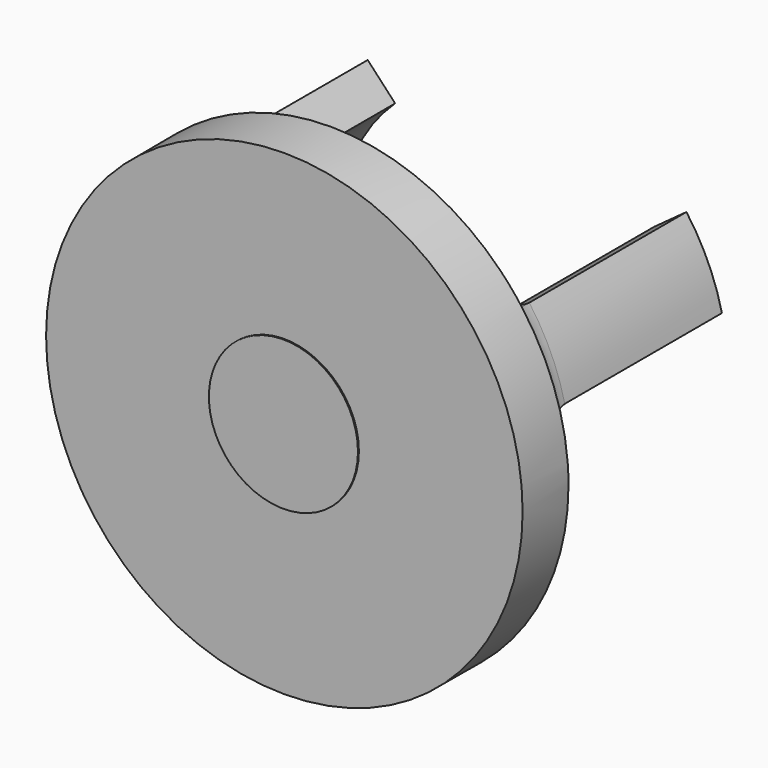
from build123d import *
from build123d import SkipClean  # not in build123d's __all__

# Parameters (mm, degrees)
F0_R          = 6.5
F1_DEPTH      = 0.1
F2_R          = 20.7743809462
F3_DEPTH      = 5
F5_DEPTH      = 25
F6_T4_DEPTH   = 18.5
F6_S5_R       = 18.6353541956
F6_T6_DEPTH   = 12
F6_S7_R       = 15.1353541956
F6_T8_DEPTH   = 12
F6_T10_ANGLE  = 23
F6_T14_DEPTH  = 18.5
F6_S15_R      = 18.6353541956
F6_T16_DEPTH  = 12
F6_S17_R      = 15.1353541956
F6_T18_DEPTH  = 12
F6_T20_ANGLE  = 23
F6_T22_ANGLE  = 23
F6_T26_DEPTH  = 18.5
F6_S27_R      = 18.6353541956
F6_T28_DEPTH  = 12
F6_S29_R      = 15.1353541956
F6_T30_DEPTH  = 12
F6_T32_ANGLE  = 23
F6_T36_DEPTH  = 18.5
F6_S37_R      = 18.6353541956
F6_T38_DEPTH  = 12
F6_S39_R      = 15.1353541956
F6_T40_DEPTH  = 12
F6_T42_ANGLE  = 23
F6_T46_DEPTH  = 18.5
F6_S47_R      = 18.6353541956
F6_T48_DEPTH  = 12
F6_S49_R      = 15.1353541956
F6_T50_DEPTH  = 12
F6_T52_ANGLE  = 23
F6_T56_DEPTH  = 18.5
F6_S57_R      = 18.6353541956
F6_T58_DEPTH  = 11
F6_S59_R      = 15.1353541956
F6_T60_DEPTH  = 11
F6_T65_ANGLE  = 45.0898559736
F6_T69_DEPTH  = 18.5
F6_S70_R      = 20.7743809462
F6_T71_DEPTH  = 12
F6_S72_R      = 18.6353541956
F6_T73_DEPTH  = 12
F6_T79_DEPTH  = 18.5
F6_S80_R      = 15.1353541956
F6_T81_DEPTH  = 12
F6_T84_ANGLE  = 51.3924387562
F6_T91_DEPTH  = 18.5
F6_S92_R      = 15.1353541956
F6_T93_DEPTH  = 12
F6_T96_ANGLE  = 51.3924387562
F6_T103_DEPTH = 18.5
F6_S104_R     = 20.7743809462
F6_T105_DEPTH = 12
F6_S106_R     = 18.6353541956
F6_T107_DEPTH = 12
F6_T110_ANGLE = 45.0898559736
F6_T117_ANGLE = 45.0898559736
F6_T121_DEPTH = 18.5
F6_S122_R     = 20.7743809462
F6_T123_DEPTH = 12
F6_S124_R     = 18.6353541956
F6_T125_DEPTH = 12
F6_T131_ANGLE = 45.0898559736
F6_T135_DEPTH = 18.5
F6_S136_R     = 20.7743809462
F6_T137_DEPTH = 12
F6_S138_R     = 18.6353541956
F6_T139_DEPTH = 12
F6_T145_DEPTH = 18.5
F6_S146_R     = 15.1353541956
F6_T147_DEPTH = 12
F6_T150_ANGLE = 51.3924387562
F6_T157_ANGLE = 51.3924387562
F6_T161_DEPTH = 18.5
F6_S162_R     = 15.1353541956
F6_T163_DEPTH = 12
F6_T169_DEPTH = 18.5
F6_S170_R     = 20.7743809462
F6_T171_DEPTH = 12
F6_S172_R     = 18.6353541956
F6_T173_DEPTH = 12
F6_T176_ANGLE = 45.0898559736
F6_T183_ANGLE = 45.0898559736
F6_T187_DEPTH = 18.5
F6_S188_R     = 20.7743809462
F6_T189_DEPTH = 11
F6_S190_R     = 18.6353541956
F6_T191_DEPTH = 11
F6_T197_DEPTH = 18.5
F6_S198_R     = 15.1353541956
F6_T199_DEPTH = 12
F6_T202_ANGLE = 51.3924387562
F6_T209_DEPTH = 18.5
F6_S210_R     = 15.1353541956
F6_T211_DEPTH = 11
F6_T214_ANGLE = 51.3924387562


# Not quite as in the source:
# - a fillet or chamfer that OpenCascade refuses, or shapes differently, is made with other operations: its cross-section is extruded or revolved along the edge and cut away or added


with BuildPart() as f1:
    # F0 (on Front) → F1 (new body)
    with BuildSketch(Plane.XZ):
        Circle(F0_R)
    extrude(amount=F1_DEPTH)

    # F2 (on Front) → F3 (join)
    with BuildSketch(Plane.XZ):
        Circle(F2_R)
    extrude(amount=-F3_DEPTH)

    # F4 (on face) → F5 (join)
    with BuildSketch(Plane.XZ):
        with BuildLine():
            Line((-10.3406240467, 11.052169061), (-12.7318587476, 13.6079461649))
            ThreePointArc((-12.7318587476, 13.6079461649), (-15.1892510411, 10.7964382464), (-17.0367859321, 7.5514469541))
            Line((-17.0367859321, 7.5514469541), (-13.8370211121, 6.1331715588))
            ThreePointArc((-13.8370211121, 6.1331715588), (-12.336481081, 8.7687046457), (-10.3406240467, 11.052169061))
        make_face()
        with BuildLine():
            Line((14.7417711971, 3.4291585849), (18.1507564459, 4.2221400303))
            ThreePointArc((18.1507564459, 4.2221400303), (16.9446153123, 7.7560581428), (15.0581378636, 10.9785659389))
            Line((15.0581378636, 10.9785659389), (12.2299929317, 8.9166260164))
            ThreePointArc((12.2299929317, 8.9166260164), (13.762161522, 6.2993536866), (14.7417711971, 3.4291585849))
        make_face()
        with BuildLine():
            ThreePointArc((-5.4188976984, -17.8300861953), (-1.7553642712, -18.5524963892), (1.9786480684, -18.5300128931))
            Line((1.9786480684, -18.5300128931), (1.6070281804, -15.0497975752))
            ThreePointArc((1.6070281804, -15.0497975752), (-1.425680441, -15.0680583323), (-4.4011471504, -14.4813276459))
            Line((-4.4011471504, -14.4813276459), (-5.4188976984, -17.8300861953))
        make_face()
    extrude(amount=-F5_DEPTH)

    # F6: fillet of radius 3 on 12 edges, made by hand


with BuildPart() as f6_tool2:
    # F6_s3 → F6_t4 (new body)
    with BuildSketch(Plane(origin=(-23.8934248319, 0, 10.5906085156), x_dir=(0, 1, 0), z_dir=(0.91421852, 0, -0.4052215415))):
        with BuildLine():
            ThreePointArc((5, -3), (5.8786796564, -0.8786796564), (8, 0))
            Line((8, 0), (8, 0.06))
            Line((8, 0.06), (4.94, 0.06))
            Line((4.94, 0.06), (4.94, -3))
            Line((4.94, -3), (5, -3))
        make_face()
    extrude(amount=F6_T4_DEPTH)

    # F6_s5 → F6_t6 (intersect, symmetric)
    with BuildSketch(Plane.XZ.offset(-6.5)):
        Circle(F6_S5_R)
    extrude(amount=F6_T6_DEPTH, both=True, mode=Mode.INTERSECT)

    # F6_s7 → F6_t8 (cut, symmetric)
    with BuildSketch(Plane.XZ.offset(-6.5)):
        Circle(F6_S7_R)
    extrude(amount=F6_T8_DEPTH, both=True, mode=Mode.SUBTRACT)


with BuildPart() as f1_1:
    add(f1.part, clean=False)

    # F6_t1: union F6_tool2
    add(f6_tool2.part)

    # F6_s9 → F6_t10 (revolve)
    with BuildSketch(Plane(origin=(0, 0, 0), x_dir=(0, 1, 0), z_dir=(0.7302220297, 0, 0.6832099145))):
        with BuildLine():
            ThreePointArc((5, 12.1353541956), (5.8786796564, 14.2566745392), (8, 15.1353541956))
            Line((8, 15.1353541956), (8, 15.1953541956))
            Line((8, 15.1953541956), (4.94, 15.1953541956))
            Line((4.94, 15.1953541956), (4.94, 12.1353541956))
            Line((4.94, 12.1353541956), (5, 12.1353541956))
        make_face()
    revolve(axis=Axis((0, 5, 0), (0, -1, 0)), revolution_arc=F6_T10_ANGLE)


with BuildPart() as f6_tool12:
    # F6_s13 → F6_t14 (new body)
    with BuildSketch(Plane(origin=(-5.2165496875, 0, 5.5755038382), x_dir=(0, 1, 0), z_dir=(-0.6832099145, 0, 0.7302220297))):
        with BuildLine():
            ThreePointArc((5, -3), (5.8786796564, -0.8786796564), (8, 0))
            Line((8, 0), (8, 0.06))
            Line((8, 0.06), (4.94, 0.06))
            Line((4.94, 0.06), (4.94, -3))
            Line((4.94, -3), (5, -3))
        make_face()
    extrude(amount=F6_T14_DEPTH)

    # F6_s15 → F6_t16 (intersect, symmetric)
    with BuildSketch(Plane.XZ.offset(-6.5)):
        Circle(F6_S15_R)
    extrude(amount=F6_T16_DEPTH, both=True, mode=Mode.INTERSECT)

    # F6_s17 → F6_t18 (cut, symmetric)
    with BuildSketch(Plane.XZ.offset(-6.5)):
        Circle(F6_S17_R)
    extrude(amount=F6_T18_DEPTH, both=True, mode=Mode.SUBTRACT)


with BuildPart() as f1_2:
    add(f1_1.part, clean=False)

    # F6_t11: union F6_tool12
    add(f6_tool12.part)

    # F6_s19 → F6_t20 (revolve)
    with BuildSketch(Plane(origin=(0, 0, 0), x_dir=(0, 1, 0), z_dir=(0.7302220297, 0, 0.6832099145))):
        with BuildLine():
            ThreePointArc((5, 20.7743809462), (6.0825599313, 19.2288089801), (7.8737997606, 18.6353541956))
            Line((7.8737997606, 18.6353541956), (7.8737997606, 18.5753541956))
            Line((7.8737997606, 18.5753541956), (5, 18.5753541956))
            Line((5, 18.5753541956), (4.94, 18.6353541956))
            ThreePointArc((4.94, 18.6353541956), (4.94, 19.7048675709), (4.9425240048, 20.7571614812))
            Line((4.9425240048, 20.7571614812), (5, 20.7743809462))
        make_face()
    revolve(axis=Axis((0, 5, 0), (0, -1, 0)), revolution_arc=F6_T20_ANGLE)

    # F6_s21 → F6_t22 (revolve)
    with BuildSketch(Plane(origin=(0, 0, 0), x_dir=(0, 1, 0), z_dir=(0.2265661273, 0, -0.9739957854))):
        with BuildLine():
            ThreePointArc((5, 20.7743809462), (6.0825599313, 19.2288089801), (7.8737997606, 18.6353541956))
            Line((7.8737997606, 18.6353541956), (7.8737997606, 18.5753541956))
            Line((7.8737997606, 18.5753541956), (5, 18.5753541956))
            Line((5, 18.5753541956), (4.94, 18.6353541956))
            ThreePointArc((4.94, 18.6353541956), (4.94, 19.7048675709), (4.9425240048, 20.7571614812))
            Line((4.9425240048, 20.7571614812), (5, 20.7743809462))
        make_face()
    revolve(axis=Axis((0, 5, 0), (0, -1, 0)), revolution_arc=F6_T22_ANGLE)


with BuildPart() as f6_tool24:
    # F6_s25 → F6_t26 (new body)
    with BuildSketch(Plane(origin=(21.118448432, 0, 15.39700863), x_dir=(0, 1, 0), z_dir=(-0.8080414091, 0, -0.5891256921))):
        with BuildLine():
            ThreePointArc((5, -3), (5.8786796564, -0.8786796564), (8, 0))
            Line((8, 0), (8, 0.06))
            Line((8, 0.06), (4.94, 0.06))
            Line((4.94, 0.06), (4.94, -3))
            Line((4.94, -3), (5, -3))
        make_face()
    extrude(amount=F6_T26_DEPTH)

    # F6_s27 → F6_t28 (intersect, symmetric)
    with BuildSketch(Plane.XZ.offset(-6.5)):
        Circle(F6_S27_R)
    extrude(amount=F6_T28_DEPTH, both=True, mode=Mode.INTERSECT)

    # F6_s29 → F6_t30 (cut, symmetric)
    with BuildSketch(Plane.XZ.offset(-6.5)):
        Circle(F6_S29_R)
    extrude(amount=F6_T30_DEPTH, both=True, mode=Mode.SUBTRACT)


with BuildPart() as f1_3:
    add(f1_2.part, clean=False)

    # F6_t23: union F6_tool24
    add(f6_tool24.part)

    # F6_s31 → F6_t32 (revolve)
    with BuildSketch(Plane(origin=(0, 0, 0), x_dir=(0, 1, 0), z_dir=(0.2265661273, 0, -0.9739957854))):
        with BuildLine():
            ThreePointArc((5, 12.1353541956), (5.8786796564, 14.2566745392), (8, 15.1353541956))
            Line((8, 15.1353541956), (8, 15.1953541956))
            Line((8, 15.1953541956), (4.94, 15.1953541956))
            Line((4.94, 15.1953541956), (4.94, 12.1353541956))
            Line((4.94, 12.1353541956), (5, 12.1353541956))
        make_face()
    revolve(axis=Axis((0, 5, 0), (0, -1, 0)), revolution_arc=F6_T32_ANGLE)


with BuildPart() as f6_tool34:
    # F6_s35 → F6_t36 (new body)
    with BuildSketch(Plane(origin=(7.4368028066, 0, 1.7299126304), x_dir=(0, 1, 0), z_dir=(0.9739957854, 0, 0.2265661273))):
        with BuildLine():
            ThreePointArc((5, -3), (5.8786796564, -0.8786796564), (8, 0))
            Line((8, 0), (8, 0.06))
            Line((8, 0.06), (4.94, 0.06))
            Line((4.94, 0.06), (4.94, -3))
            Line((4.94, -3), (5, -3))
        make_face()
    extrude(amount=F6_T36_DEPTH)

    # F6_s37 → F6_t38 (intersect, symmetric)
    with BuildSketch(Plane.XZ.offset(-6.5)):
        Circle(F6_S37_R)
    extrude(amount=F6_T38_DEPTH, both=True, mode=Mode.INTERSECT)

    # F6_s39 → F6_t40 (cut, symmetric)
    with BuildSketch(Plane.XZ.offset(-6.5)):
        Circle(F6_S39_R)
    extrude(amount=F6_T40_DEPTH, both=True, mode=Mode.SUBTRACT)


with BuildPart() as f1_4:
    add(f1_3.part, clean=False)

    # F6_t33: union F6_tool34
    add(f6_tool34.part)

    # F6_s41 → F6_t42 (revolve)
    with BuildSketch(Plane(origin=(0, 0, 0), x_dir=(0, 1, 0), z_dir=(-0.956788157, 0, 0.2907858709))):
        with BuildLine():
            ThreePointArc((5, 20.7743809462), (6.0825599313, 19.2288089801), (7.8737997606, 18.6353541956))
            Line((7.8737997606, 18.6353541956), (7.8737997606, 18.5753541956))
            Line((7.8737997606, 18.5753541956), (5, 18.5753541956))
            Line((5, 18.5753541956), (4.94, 18.6353541956))
            ThreePointArc((4.94, 18.6353541956), (4.94, 19.7048675709), (4.9425240048, 20.7571614812))
            Line((4.9425240048, 20.7571614812), (5, 20.7743809462))
        make_face()
    revolve(axis=Axis((0, 5, 0), (0, -1, 0)), revolution_arc=F6_T42_ANGLE)


with BuildPart() as f6_tool44:
    # F6_s45 → F6_t46 (new body)
    with BuildSketch(Plane(origin=(-2.220253119, 0, -7.3054164686), x_dir=(0, 1, 0), z_dir=(-0.2907858709, 0, -0.956788157))):
        with BuildLine():
            ThreePointArc((5, -3), (5.8786796564, -0.8786796564), (8, 0))
            Line((8, 0), (8, 0.06))
            Line((8, 0.06), (4.94, 0.06))
            Line((4.94, 0.06), (4.94, -3))
            Line((4.94, -3), (5, -3))
        make_face()
    extrude(amount=F6_T46_DEPTH)

    # F6_s47 → F6_t48 (intersect, symmetric)
    with BuildSketch(Plane.XZ.offset(-6.5)):
        Circle(F6_S47_R)
    extrude(amount=F6_T48_DEPTH, both=True, mode=Mode.INTERSECT)

    # F6_s49 → F6_t50 (cut, symmetric)
    with BuildSketch(Plane.XZ.offset(-6.5)):
        Circle(F6_S49_R)
    extrude(amount=F6_T50_DEPTH, both=True, mode=Mode.SUBTRACT)


with BuildPart() as f1_5:
    add(f1_4.part, clean=False)

    # F6_t43: union F6_tool44
    add(f6_tool44.part)

    # F6_s51 → F6_t52 (revolve)
    with BuildSketch(Plane(origin=(0, 0, 0), x_dir=(0, 1, 0), z_dir=(-0.956788157, 0, 0.2907858709))):
        with BuildLine():
            ThreePointArc((5, 12.1353541956), (5.8786796564, 14.2566745392), (8, 15.1353541956))
            Line((8, 15.1353541956), (8, 15.1953541956))
            Line((8, 15.1953541956), (4.94, 15.1953541956))
            Line((4.94, 15.1953541956), (4.94, 12.1353541956))
            Line((4.94, 12.1353541956), (5, 12.1353541956))
        make_face()
    with SkipClean():  # cleaning this boolean's faces spoils the solid; the shape is the same uncleaned
        revolve(axis=Axis((0, 5, 0), (0, -1, 0)), revolution_arc=F6_T52_ANGLE)


with BuildPart() as f6_tool54:
    # F6_s55 → F6_t56 (new body)
    with BuildSketch(Plane(origin=(2.7749763999, 0, -25.9876171457), x_dir=(0, 1, 0), z_dir=(-0.1061771109, 0, 0.9943472337))):
        with BuildLine():
            ThreePointArc((5, -3), (5.8786796564, -0.8786796564), (8, 0))
            Line((8, 0), (8, 0.06))
            Line((8, 0.06), (4.94, 0.06))
            Line((4.94, 0.06), (4.94, -3))
            Line((4.94, -3), (5, -3))
        make_face()
    extrude(amount=F6_T56_DEPTH)

    # F6_s57 → F6_t58 (intersect, symmetric)
    with BuildSketch(Plane.XZ.offset(-6.5)):
        Circle(F6_S57_R)
    extrude(amount=F6_T58_DEPTH, both=True, mode=Mode.INTERSECT)

    # F6_s59 → F6_t60 (cut, symmetric)
    with BuildSketch(Plane.XZ.offset(-6.5)):
        Circle(F6_S59_R)
    extrude(amount=F6_T60_DEPTH, both=True, mode=Mode.SUBTRACT)


with BuildPart() as f1_6:
    add(f1_5.part, clean=False)

    # F6_t53: union F6_tool54
    add(f6_tool54.part)


with BuildPart() as f6_tool63:
    # F6_s64 → F6_t65 (revolve)
    with BuildSketch(Plane(origin=(0, 0, 0), x_dir=(0, 1, 0), z_dir=(0.7302220297, 0, 0.6832099145))):
        with BuildLine():
            ThreePointArc((5, 20.7743809462), (6.0825599313, 19.2288089801), (7.8737997606, 18.6353541956))
            Line((7.8737997606, 18.6353541956), (7.8737997606, 18.5753541956))
            Line((7.8737997606, 18.5753541956), (5, 18.5753541956))
            Line((5, 18.5753541956), (4.94, 18.6353541956))
            ThreePointArc((4.94, 18.6353541956), (4.94, 19.7048675709), (4.9425240048, 20.7571614812))
            Line((4.9425240048, 20.7571614812), (5, 20.7743809462))
        make_face()
    revolve(axis=Axis((0, 5, 0), (0, -1, 0)), revolution_arc=F6_T65_ANGLE)

    split(bisect_by=Plane(origin=(0, 0, 0), x_dir=(0, 1, 0), z_dir=(-0.4052215415, 0, -0.91421852)), keep=Keep.TOP)


with BuildPart() as f6_tool67:
    # F6_s68 → F6_t69 (new body)
    with BuildSketch(Plane(origin=(-23.8934248319, 0, 10.5906085156), x_dir=(0, 1, 0), z_dir=(0.91421852, 0, -0.4052215415))):
        with BuildLine():
            ThreePointArc((5, -3), (5.8786796564, -0.8786796564), (8, 0))
            Line((8, 0), (8, 0.06))
            Line((8, 0.06), (4.94, 0.06))
            Line((4.94, 0.06), (4.94, -3))
            Line((4.94, -3), (5, -3))
        make_face()
    extrude(amount=F6_T69_DEPTH)

    # F6_s70 → F6_t71 (intersect, symmetric)
    with BuildSketch(Plane.XZ.offset(-6.5)):
        Circle(F6_S70_R)
    extrude(amount=F6_T71_DEPTH, both=True, mode=Mode.INTERSECT)

    # F6_s72 → F6_t73 (cut, symmetric)
    with BuildSketch(Plane.XZ.offset(-6.5)):
        Circle(F6_S72_R)
    extrude(amount=F6_T73_DEPTH, both=True, mode=Mode.SUBTRACT)


with BuildPart() as f6_tool63_1:
    add(f6_tool63.part, clean=False)

    # F6_t74: intersect F6_tool67
    add(f6_tool67.part, mode=Mode.INTERSECT)


with BuildPart() as f1_7:
    add(f1_6.part, clean=False)

    # F6_t61: union F6_tool63
    add(f6_tool63_1.part)


with BuildPart() as f6_tool77:
    # F6_s78 → F6_t79 (new body)
    with BuildSketch(Plane(origin=(-23.8934248319, 0, 10.5906085156), x_dir=(0, 1, 0), z_dir=(0.91421852, 0, -0.4052215415))):
        with BuildLine():
            ThreePointArc((5, -3), (5.8786796564, -0.8786796564), (8, 0))
            Line((8, 0), (8, 0.06))
            Line((8, 0.06), (4.94, 0.06))
            Line((4.94, 0.06), (4.94, -3))
            Line((4.94, -3), (5, -3))
        make_face()
    extrude(amount=F6_T79_DEPTH)

    # F6_s80 → F6_t81 (intersect, symmetric)
    with BuildSketch(Plane.XZ.offset(-6.5)):
        Circle(F6_S80_R)
    extrude(amount=F6_T81_DEPTH, both=True, mode=Mode.INTERSECT)


with BuildPart() as f6_tool82:
    # F6_s83 → F6_t84 (revolve)
    with BuildSketch(Plane(origin=(0, 0, 0), x_dir=(0, 1, 0), z_dir=(0.7302220297, 0, 0.6832099145))):
        with BuildLine():
            ThreePointArc((5, 12.1353541956), (5.8786796564, 14.2566745392), (8, 15.1353541956))
            Line((8, 15.1353541956), (8, 15.1953541956))
            Line((8, 15.1953541956), (4.94, 15.1953541956))
            Line((4.94, 15.1953541956), (4.94, 12.1353541956))
            Line((4.94, 12.1353541956), (5, 12.1353541956))
        make_face()
    revolve(axis=Axis((0, 5, 0), (0, -1, 0)), revolution_arc=F6_T84_ANGLE)

    split(bisect_by=Plane(origin=(0, 0, 0), x_dir=(0, 1, 0), z_dir=(-0.4052215415, 0, -0.91421852)), keep=Keep.TOP)


with BuildPart() as f6_tool77_1:
    add(f6_tool77.part, clean=False)

    # F6_t86: intersect F6_tool82
    add(f6_tool82.part, mode=Mode.INTERSECT)


with BuildPart() as f1_8:
    add(f1_7.part, clean=False)

    # F6_t75: union F6_tool77
    add(f6_tool77_1.part)


with BuildPart() as f6_tool89:
    # F6_s90 → F6_t91 (new body)
    with BuildSketch(Plane(origin=(-5.2165496875, 0, 5.5755038382), x_dir=(0, 1, 0), z_dir=(-0.6832099145, 0, 0.7302220297))):
        with BuildLine():
            ThreePointArc((5, -3), (5.8786796564, -0.8786796564), (8, 0))
            Line((8, 0), (8, 0.06))
            Line((8, 0.06), (4.94, 0.06))
            Line((4.94, 0.06), (4.94, -3))
            Line((4.94, -3), (5, -3))
        make_face()
    extrude(amount=F6_T91_DEPTH)

    # F6_s92 → F6_t93 (intersect, symmetric)
    with BuildSketch(Plane.XZ.offset(-6.5)):
        Circle(F6_S92_R)
    extrude(amount=F6_T93_DEPTH, both=True, mode=Mode.INTERSECT)


with BuildPart() as f6_tool94:
    # F6_s95 → F6_t96 (revolve)
    with BuildSketch(Plane(origin=(0, 0, 0), x_dir=(0, 1, 0), z_dir=(0.9672564562, 0, 0.2538010007))):
        with BuildLine():
            ThreePointArc((5, 12.1353541956), (5.8786796564, 14.2566745392), (8, 15.1353541956))
            Line((8, 15.1353541956), (8, 15.1953541956))
            Line((8, 15.1953541956), (4.94, 15.1953541956))
            Line((4.94, 15.1953541956), (4.94, 12.1353541956))
            Line((4.94, 12.1353541956), (5, 12.1353541956))
        make_face()
    revolve(axis=Axis((0, 5, 0), (0, -1, 0)), revolution_arc=F6_T96_ANGLE)

    split(bisect_by=Plane(origin=(0, 0, 0), x_dir=(0, 1, 0), z_dir=(0.7302220297, 0, 0.6832099145)), keep=Keep.TOP)


with BuildPart() as f6_tool89_1:
    add(f6_tool89.part, clean=False)

    # F6_t98: intersect F6_tool94
    add(f6_tool94.part, mode=Mode.INTERSECT)


with BuildPart() as f1_9:
    add(f1_8.part, clean=False)

    # F6_t87: union F6_tool89
    add(f6_tool89_1.part)


with BuildPart() as f6_tool101:
    # F6_s102 → F6_t103 (new body)
    with BuildSketch(Plane(origin=(-5.2165496875, 0, 5.5755038382), x_dir=(0, 1, 0), z_dir=(-0.6832099145, 0, 0.7302220297))):
        with BuildLine():
            ThreePointArc((5, -3), (5.8786796564, -0.8786796564), (8, 0))
            Line((8, 0), (8, 0.06))
            Line((8, 0.06), (4.94, 0.06))
            Line((4.94, 0.06), (4.94, -3))
            Line((4.94, -3), (5, -3))
        make_face()
    extrude(amount=F6_T103_DEPTH)

    # F6_s104 → F6_t105 (intersect, symmetric)
    with BuildSketch(Plane.XZ.offset(-6.5)):
        Circle(F6_S104_R)
    extrude(amount=F6_T105_DEPTH, both=True, mode=Mode.INTERSECT)

    # F6_s106 → F6_t107 (cut, symmetric)
    with BuildSketch(Plane.XZ.offset(-6.5)):
        Circle(F6_S106_R)
    extrude(amount=F6_T107_DEPTH, both=True, mode=Mode.SUBTRACT)


with BuildPart() as f6_tool108:
    # F6_s109 → F6_t110 (revolve)
    with BuildSketch(Plane(origin=(0, 0, 0), x_dir=(0, 1, 0), z_dir=(0.9335483161, 0, 0.3584515889))):
        with BuildLine():
            ThreePointArc((5, 20.7743809462), (6.0825599313, 19.2288089801), (7.8737997606, 18.6353541956))
            Line((7.8737997606, 18.6353541956), (7.8737997606, 18.5753541956))
            Line((7.8737997606, 18.5753541956), (5, 18.5753541956))
            Line((5, 18.5753541956), (4.94, 18.6353541956))
            ThreePointArc((4.94, 18.6353541956), (4.94, 19.7048675709), (4.9425240048, 20.7571614812))
            Line((4.9425240048, 20.7571614812), (5, 20.7743809462))
        make_face()
    revolve(axis=Axis((0, 5, 0), (0, -1, 0)), revolution_arc=F6_T110_ANGLE)

    split(bisect_by=Plane(origin=(0, 0, 0), x_dir=(0, 1, 0), z_dir=(0.7302220297, 0, 0.6832099145)), keep=Keep.TOP)


with BuildPart() as f6_tool101_1:
    add(f6_tool101.part, clean=False)

    # F6_t112: intersect F6_tool108
    add(f6_tool108.part, mode=Mode.INTERSECT)


with BuildPart() as f1_10:
    add(f1_9.part, clean=False)

    # F6_t99: union F6_tool101
    add(f6_tool101_1.part)


with BuildPart() as f6_tool115:
    # F6_s116 → F6_t117 (revolve)
    with BuildSketch(Plane(origin=(0, 0, 0), x_dir=(0, 1, 0), z_dir=(-0.156345976, 0, -0.9877023518))):
        with BuildLine():
            ThreePointArc((5, 20.7743809462), (6.0825599313, 19.2288089801), (7.8737997606, 18.6353541956))
            Line((7.8737997606, 18.6353541956), (7.8737997606, 18.5753541956))
            Line((7.8737997606, 18.5753541956), (5, 18.5753541956))
            Line((5, 18.5753541956), (4.94, 18.6353541956))
            ThreePointArc((4.94, 18.6353541956), (4.94, 19.7048675709), (4.9425240048, 20.7571614812))
            Line((4.9425240048, 20.7571614812), (5, 20.7743809462))
        make_face()
    revolve(axis=Axis((0, 5, 0), (0, -1, 0)), revolution_arc=F6_T117_ANGLE)

    split(bisect_by=Plane(origin=(0, 0, 0), x_dir=(0, 1, 0), z_dir=(0.2265661273, 0, -0.9739957854)), keep=Keep.TOP)


with BuildPart() as f6_tool119:
    # F6_s120 → F6_t121 (new body)
    with BuildSketch(Plane(origin=(7.4368028066, 0, 1.7299126304), x_dir=(0, 1, 0), z_dir=(0.9739957854, 0, 0.2265661273))):
        with BuildLine():
            ThreePointArc((5, -3), (5.8786796564, -0.8786796564), (8, 0))
            Line((8, 0), (8, 0.06))
            Line((8, 0.06), (4.94, 0.06))
            Line((4.94, 0.06), (4.94, -3))
            Line((4.94, -3), (5, -3))
        make_face()
    extrude(amount=F6_T121_DEPTH)

    # F6_s122 → F6_t123 (intersect, symmetric)
    with BuildSketch(Plane.XZ.offset(-6.5)):
        Circle(F6_S122_R)
    extrude(amount=F6_T123_DEPTH, both=True, mode=Mode.INTERSECT)

    # F6_s124 → F6_t125 (cut, symmetric)
    with BuildSketch(Plane.XZ.offset(-6.5)):
        Circle(F6_S124_R)
    extrude(amount=F6_T125_DEPTH, both=True, mode=Mode.SUBTRACT)


with BuildPart() as f6_tool115_1:
    add(f6_tool115.part, clean=False)

    # F6_t126: intersect F6_tool119
    add(f6_tool119.part, mode=Mode.INTERSECT)


with BuildPart() as f1_11:
    add(f1_10.part, clean=False)

    # F6_t113: union F6_tool115
    add(f6_tool115_1.part)


with BuildPart() as f6_tool129:
    # F6_s130 → F6_t131 (revolve)
    with BuildSketch(Plane(origin=(0, 0, 0), x_dir=(0, 1, 0), z_dir=(0.2265661273, 0, -0.9739957854))):
        with BuildLine():
            ThreePointArc((5, 20.7743809462), (6.0825599313, 19.2288089801), (7.8737997606, 18.6353541956))
            Line((7.8737997606, 18.6353541956), (7.8737997606, 18.5753541956))
            Line((7.8737997606, 18.5753541956), (5, 18.5753541956))
            Line((5, 18.5753541956), (4.94, 18.6353541956))
            ThreePointArc((4.94, 18.6353541956), (4.94, 19.7048675709), (4.9425240048, 20.7571614812))
            Line((4.9425240048, 20.7571614812), (5, 20.7743809462))
        make_face()
    revolve(axis=Axis((0, 5, 0), (0, -1, 0)), revolution_arc=F6_T131_ANGLE)

    split(bisect_by=Plane(origin=(0, 0, 0), x_dir=(0, 1, 0), z_dir=(-0.5891256921, 0, 0.8080414091)), keep=Keep.TOP)


with BuildPart() as f6_tool133:
    # F6_s134 → F6_t135 (new body)
    with BuildSketch(Plane(origin=(21.118448432, 0, 15.39700863), x_dir=(0, 1, 0), z_dir=(-0.8080414091, 0, -0.5891256921))):
        with BuildLine():
            ThreePointArc((5, -3), (5.8786796564, -0.8786796564), (8, 0))
            Line((8, 0), (8, 0.06))
            Line((8, 0.06), (4.94, 0.06))
            Line((4.94, 0.06), (4.94, -3))
            Line((4.94, -3), (5, -3))
        make_face()
    extrude(amount=F6_T135_DEPTH)

    # F6_s136 → F6_t137 (intersect, symmetric)
    with BuildSketch(Plane.XZ.offset(-6.5)):
        Circle(F6_S136_R)
    extrude(amount=F6_T137_DEPTH, both=True, mode=Mode.INTERSECT)

    # F6_s138 → F6_t139 (cut, symmetric)
    with BuildSketch(Plane.XZ.offset(-6.5)):
        Circle(F6_S138_R)
    extrude(amount=F6_T139_DEPTH, both=True, mode=Mode.SUBTRACT)


with BuildPart() as f6_tool129_1:
    add(f6_tool129.part, clean=False)

    # F6_t140: intersect F6_tool133
    add(f6_tool133.part, mode=Mode.INTERSECT)


with BuildPart() as f1_12:
    add(f1_11.part, clean=False)

    # F6_t127: union F6_tool129
    add(f6_tool129_1.part)


with BuildPart() as f6_tool143:
    # F6_s144 → F6_t145 (new body)
    with BuildSketch(Plane(origin=(21.118448432, 0, 15.39700863), x_dir=(0, 1, 0), z_dir=(-0.8080414091, 0, -0.5891256921))):
        with BuildLine():
            ThreePointArc((5, -3), (5.8786796564, -0.8786796564), (8, 0))
            Line((8, 0), (8, 0.06))
            Line((8, 0.06), (4.94, 0.06))
            Line((4.94, 0.06), (4.94, -3))
            Line((4.94, -3), (5, -3))
        make_face()
    extrude(amount=F6_T145_DEPTH)

    # F6_s146 → F6_t147 (intersect, symmetric)
    with BuildSketch(Plane.XZ.offset(-6.5)):
        Circle(F6_S146_R)
    extrude(amount=F6_T147_DEPTH, both=True, mode=Mode.INTERSECT)


with BuildPart() as f6_tool148:
    # F6_s149 → F6_t150 (revolve)
    with BuildSketch(Plane(origin=(0, 0, 0), x_dir=(0, 1, 0), z_dir=(0.2265661273, 0, -0.9739957854))):
        with BuildLine():
            ThreePointArc((5, 12.1353541956), (5.8786796564, 14.2566745392), (8, 15.1353541956))
            Line((8, 15.1353541956), (8, 15.1953541956))
            Line((8, 15.1953541956), (4.94, 15.1953541956))
            Line((4.94, 15.1953541956), (4.94, 12.1353541956))
            Line((4.94, 12.1353541956), (5, 12.1353541956))
        make_face()
    revolve(axis=Axis((0, 5, 0), (0, -1, 0)), revolution_arc=F6_T150_ANGLE)

    split(bisect_by=Plane(origin=(0, 0, 0), x_dir=(0, 1, 0), z_dir=(-0.5891256921, 0, 0.8080414091)), keep=Keep.TOP)


with BuildPart() as f6_tool143_1:
    add(f6_tool143.part, clean=False)

    # F6_t152: intersect F6_tool148
    add(f6_tool148.part, mode=Mode.INTERSECT)


with BuildPart() as f1_13:
    add(f1_12.part, clean=False)

    # F6_t141: union F6_tool143
    add(f6_tool143_1.part)


with BuildPart() as f6_tool155:
    # F6_s156 → F6_t157 (revolve)
    with BuildSketch(Plane(origin=(0, 0, 0), x_dir=(0, 1, 0), z_dir=(-0.263830114, 0, -0.9645691634))):
        with BuildLine():
            ThreePointArc((5, 12.1353541956), (5.8786796564, 14.2566745392), (8, 15.1353541956))
            Line((8, 15.1353541956), (8, 15.1953541956))
            Line((8, 15.1953541956), (4.94, 15.1953541956))
            Line((4.94, 15.1953541956), (4.94, 12.1353541956))
            Line((4.94, 12.1353541956), (5, 12.1353541956))
        make_face()
    revolve(axis=Axis((0, 5, 0), (0, -1, 0)), revolution_arc=F6_T157_ANGLE)

    split(bisect_by=Plane(origin=(0, 0, 0), x_dir=(0, 1, 0), z_dir=(0.2265661273, 0, -0.9739957854)), keep=Keep.TOP)


with BuildPart() as f6_tool159:
    # F6_s160 → F6_t161 (new body)
    with BuildSketch(Plane(origin=(7.4368028066, 0, 1.7299126304), x_dir=(0, 1, 0), z_dir=(0.9739957854, 0, 0.2265661273))):
        with BuildLine():
            ThreePointArc((5, -3), (5.8786796564, -0.8786796564), (8, 0))
            Line((8, 0), (8, 0.06))
            Line((8, 0.06), (4.94, 0.06))
            Line((4.94, 0.06), (4.94, -3))
            Line((4.94, -3), (5, -3))
        make_face()
    extrude(amount=F6_T161_DEPTH)

    # F6_s162 → F6_t163 (intersect, symmetric)
    with BuildSketch(Plane.XZ.offset(-6.5)):
        Circle(F6_S162_R)
    extrude(amount=F6_T163_DEPTH, both=True, mode=Mode.INTERSECT)


with BuildPart() as f6_tool155_1:
    add(f6_tool155.part, clean=False)

    # F6_t164: intersect F6_tool159
    add(f6_tool159.part, mode=Mode.INTERSECT)


with BuildPart() as f1_14:
    add(f1_13.part, clean=False)

    # F6_t153: union F6_tool155
    add(f6_tool155_1.part)


with BuildPart() as f6_tool167:
    # F6_s168 → F6_t169 (new body)
    with BuildSketch(Plane(origin=(-2.220253119, 0, -7.3054164686), x_dir=(0, 1, 0), z_dir=(-0.2907858709, 0, -0.956788157))):
        with BuildLine():
            ThreePointArc((5, -3), (5.8786796564, -0.8786796564), (8, 0))
            Line((8, 0), (8, 0.06))
            Line((8, 0.06), (4.94, 0.06))
            Line((4.94, 0.06), (4.94, -3))
            Line((4.94, -3), (5, -3))
        make_face()
    extrude(amount=F6_T169_DEPTH)

    # F6_s170 → F6_t171 (intersect, symmetric)
    with BuildSketch(Plane.XZ.offset(-6.5)):
        Circle(F6_S170_R)
    extrude(amount=F6_T171_DEPTH, both=True, mode=Mode.INTERSECT)

    # F6_s172 → F6_t173 (cut, symmetric)
    with BuildSketch(Plane.XZ.offset(-6.5)):
        Circle(F6_S172_R)
    extrude(amount=F6_T173_DEPTH, both=True, mode=Mode.SUBTRACT)


with BuildPart() as f6_tool174:
    # F6_s175 → F6_t176 (revolve)
    with BuildSketch(Plane(origin=(0, 0, 0), x_dir=(0, 1, 0), z_dir=(-0.77720234, 0, 0.6292507629))):
        with BuildLine():
            ThreePointArc((5, 20.7743809462), (6.0825599313, 19.2288089801), (7.8737997606, 18.6353541956))
            Line((7.8737997606, 18.6353541956), (7.8737997606, 18.5753541956))
            Line((7.8737997606, 18.5753541956), (5, 18.5753541956))
            Line((5, 18.5753541956), (4.94, 18.6353541956))
            ThreePointArc((4.94, 18.6353541956), (4.94, 19.7048675709), (4.9425240048, 20.7571614812))
            Line((4.9425240048, 20.7571614812), (5, 20.7743809462))
        make_face()
    revolve(axis=Axis((0, 5, 0), (0, -1, 0)), revolution_arc=F6_T176_ANGLE)

    split(bisect_by=Plane(origin=(0, 0, 0), x_dir=(0, 1, 0), z_dir=(-0.956788157, 0, 0.2907858709)), keep=Keep.TOP)


with BuildPart() as f6_tool167_1:
    add(f6_tool167.part, clean=False)

    # F6_t178: intersect F6_tool174
    add(f6_tool174.part, mode=Mode.INTERSECT)


with BuildPart() as f1_15:
    add(f1_14.part, clean=False)

    # F6_t165: union F6_tool167
    add(f6_tool167_1.part)


with BuildPart() as f6_tool181:
    # F6_s182 → F6_t183 (revolve)
    with BuildSketch(Plane(origin=(0, 0, 0), x_dir=(0, 1, 0), z_dir=(-0.956788157, 0, 0.2907858709))):
        with BuildLine():
            ThreePointArc((5, 20.7743809462), (6.0825599313, 19.2288089801), (7.8737997606, 18.6353541956))
            Line((7.8737997606, 18.6353541956), (7.8737997606, 18.5753541956))
            Line((7.8737997606, 18.5753541956), (5, 18.5753541956))
            Line((5, 18.5753541956), (4.94, 18.6353541956))
            ThreePointArc((4.94, 18.6353541956), (4.94, 19.7048675709), (4.9425240048, 20.7571614812))
            Line((4.9425240048, 20.7571614812), (5, 20.7743809462))
        make_face()
    revolve(axis=Axis((0, 5, 0), (0, -1, 0)), revolution_arc=F6_T183_ANGLE)

    split(bisect_by=Plane(origin=(0, 0, 0), x_dir=(0, 1, 0), z_dir=(0.9943472337, 0, 0.1061771109)), keep=Keep.TOP)


with BuildPart() as f6_tool185:
    # F6_s186 → F6_t187 (new body)
    with BuildSketch(Plane(origin=(2.7749763999, 0, -25.9876171457), x_dir=(0, 1, 0), z_dir=(-0.1061771109, 0, 0.9943472337))):
        with BuildLine():
            ThreePointArc((5, -3), (5.8786796564, -0.8786796564), (8, 0))
            Line((8, 0), (8, 0.06))
            Line((8, 0.06), (4.94, 0.06))
            Line((4.94, 0.06), (4.94, -3))
            Line((4.94, -3), (5, -3))
        make_face()
    extrude(amount=F6_T187_DEPTH)

    # F6_s188 → F6_t189 (intersect, symmetric)
    with BuildSketch(Plane.XZ.offset(-6.5)):
        Circle(F6_S188_R)
    extrude(amount=F6_T189_DEPTH, both=True, mode=Mode.INTERSECT)

    # F6_s190 → F6_t191 (cut, symmetric)
    with BuildSketch(Plane.XZ.offset(-6.5)):
        Circle(F6_S190_R)
    extrude(amount=F6_T191_DEPTH, both=True, mode=Mode.SUBTRACT)


with BuildPart() as f6_tool181_1:
    add(f6_tool181.part, clean=False)

    # F6_t192: intersect F6_tool185
    add(f6_tool185.part, mode=Mode.INTERSECT)


with BuildPart() as f1_16:
    add(f1_15.part, clean=False)

    # F6_t179: union F6_tool181
    add(f6_tool181_1.part)


with BuildPart() as f6_tool195:
    # F6_s196 → F6_t197 (new body)
    with BuildSketch(Plane(origin=(-2.220253119, 0, -7.3054164686), x_dir=(0, 1, 0), z_dir=(-0.2907858709, 0, -0.956788157))):
        with BuildLine():
            ThreePointArc((5, -3), (5.8786796564, -0.8786796564), (8, 0))
            Line((8, 0), (8, 0.06))
            Line((8, 0.06), (4.94, 0.06))
            Line((4.94, 0.06), (4.94, -3))
            Line((4.94, -3), (5, -3))
        make_face()
    extrude(amount=F6_T197_DEPTH)

    # F6_s198 → F6_t199 (intersect, symmetric)
    with BuildSketch(Plane.XZ.offset(-6.5)):
        Circle(F6_S198_R)
    extrude(amount=F6_T199_DEPTH, both=True, mode=Mode.INTERSECT)


with BuildPart() as f6_tool200:
    # F6_s201 → F6_t202 (revolve)
    with BuildSketch(Plane(origin=(0, 0, 0), x_dir=(0, 1, 0), z_dir=(-0.7034263422, 0, 0.7107681627))):
        with BuildLine():
            ThreePointArc((5, 12.1353541956), (5.8786796564, 14.2566745392), (8, 15.1353541956))
            Line((8, 15.1353541956), (8, 15.1953541956))
            Line((8, 15.1953541956), (4.94, 15.1953541956))
            Line((4.94, 15.1953541956), (4.94, 12.1353541956))
            Line((4.94, 12.1353541956), (5, 12.1353541956))
        make_face()
    revolve(axis=Axis((0, 5, 0), (0, -1, 0)), revolution_arc=F6_T202_ANGLE)

    split(bisect_by=Plane(origin=(0, 0, 0), x_dir=(0, 1, 0), z_dir=(-0.956788157, 0, 0.2907858709)), keep=Keep.TOP)


with BuildPart() as f6_tool195_1:
    add(f6_tool195.part, clean=False)

    # F6_t204: intersect F6_tool200
    add(f6_tool200.part, mode=Mode.INTERSECT)


with BuildPart() as f1_17:
    add(f1_16.part, clean=False)

    # F6_t193: union F6_tool195
    add(f6_tool195_1.part)


with BuildPart() as f6_tool207:
    # F6_s208 → F6_t209 (new body)
    with BuildSketch(Plane(origin=(2.7749763999, 0, -25.9876171457), x_dir=(0, 1, 0), z_dir=(-0.1061771109, 0, 0.9943472337))):
        with BuildLine():
            ThreePointArc((5, -3), (5.8786796564, -0.8786796564), (8, 0))
            Line((8, 0), (8, 0.06))
            Line((8, 0.06), (4.94, 0.06))
            Line((4.94, 0.06), (4.94, -3))
            Line((4.94, -3), (5, -3))
        make_face()
    extrude(amount=F6_T209_DEPTH)

    # F6_s210 → F6_t211 (intersect, symmetric)
    with BuildSketch(Plane.XZ.offset(-6.5)):
        Circle(F6_S210_R)
    extrude(amount=F6_T211_DEPTH, both=True, mode=Mode.INTERSECT)


with BuildPart() as f6_tool212:
    # F6_s213 → F6_t214 (revolve)
    with BuildSketch(Plane(origin=(0, 0, 0), x_dir=(0, 1, 0), z_dir=(-0.956788157, 0, 0.2907858709))):
        with BuildLine():
            ThreePointArc((5, 12.1353541956), (5.8786796564, 14.2566745392), (8, 15.1353541956))
            Line((8, 15.1353541956), (8, 15.1953541956))
            Line((8, 15.1953541956), (4.94, 15.1953541956))
            Line((4.94, 15.1953541956), (4.94, 12.1353541956))
            Line((4.94, 12.1353541956), (5, 12.1353541956))
        make_face()
    revolve(axis=Axis((0, 5, 0), (0, -1, 0)), revolution_arc=F6_T214_ANGLE)

    split(bisect_by=Plane(origin=(0, 0, 0), x_dir=(0, 1, 0), z_dir=(0.9943472337, 0, 0.1061771109)), keep=Keep.TOP)


with BuildPart() as f6_tool207_1:
    add(f6_tool207.part, clean=False)

    # F6_t216: intersect F6_tool212
    add(f6_tool212.part, mode=Mode.INTERSECT)


with BuildPart() as f1_18:
    add(f1_17.part, clean=False)

    # F6_t205: union F6_tool207
    add(f6_tool207_1.part)


solid = f1_18.part
